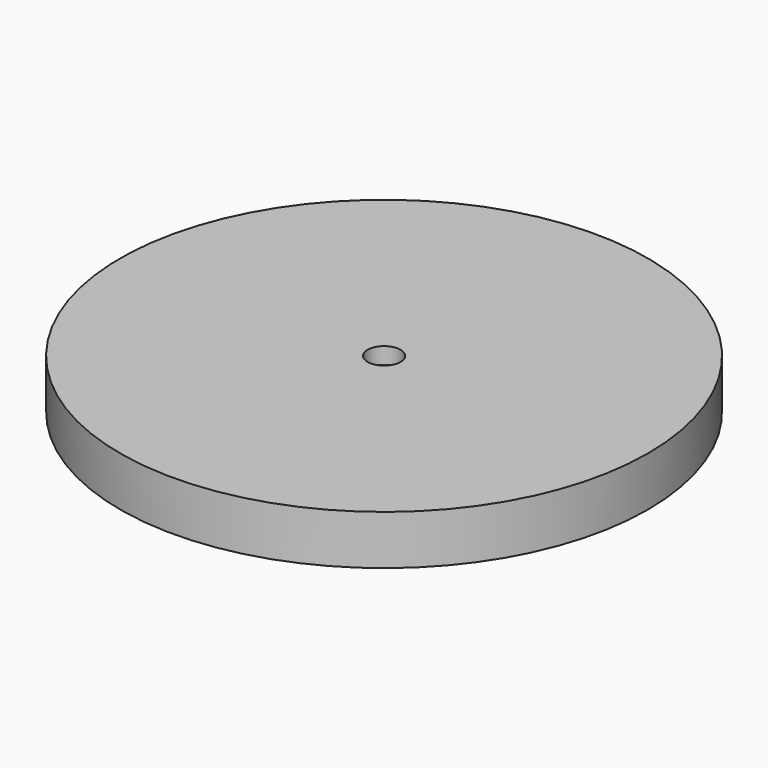
from build123d import *

# Parameters (mm, degrees)
F0_R     = 101.6
F1_DEPTH = 19.05
F2_R     = 6.35
F3_DEPTH = 6.35


# Not quite as in the source:
# - a length typed as a fraction of an inch, garbled in the dataset ("3 / 203.2 mm" for 3/8 in), is restored


with BuildPart() as f1:
    # F0 (on Top) → F1 (new body)
    with BuildSketch(Plane.XY):
        Circle(F0_R)
    extrude(amount=F1_DEPTH)

    # F2 (on face) → F3 (cut)
    with BuildSketch(Plane.XY.offset(19.05)):
        Circle(F2_R)
    extrude(amount=-F3_DEPTH, mode=Mode.SUBTRACT)


solid = f1.part
